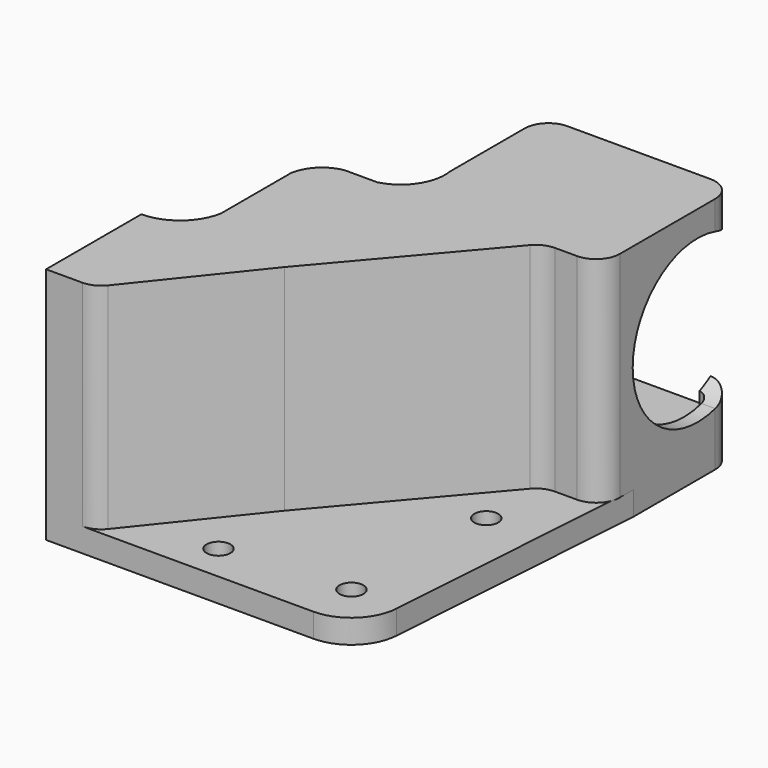
from build123d import *

# Parameters (mm, degrees)
F1_DEPTH    = 57.15
F2_T        = 3.683
F2_T3_DEPTH = 64.516
F4_DEPTH    = 25.4
F6_DEPTH    = 6.35
F7_R        = 3.175
F8_DEPTH    = 25.4
F10_DEPTH   = 56.642


# Not quite as in the source:
# - a shell that OpenCascade refuses in one call is made with other operations: the cavity is built on its own and cut out


with BuildPart() as f1:
    # F0 (on Top) → F1 (new body)
    with BuildSketch(Plane.XY):
        with BuildLine():
            ThreePointArc((33.7229068752, -2.2373507569), (35.8958962, -0.5864150612), (38.5611520326, 0))
            Line((38.5611520326, 0), (44.45, 0))
            ThreePointArc((44.45, 0), (48.9401280605, 1.8598719395), (50.8, 6.35))
            Line((50.8, 6.35), (50.8, 38.1))
            ThreePointArc((50.8, 38.1), (48.9401280605, 42.5901280605), (44.45, 44.45))
            Line((44.45, 44.45), (6.35, 44.45))
            ThreePointArc((6.35, 44.45), (1.8598719395, 42.5901280605), (0, 38.1))
            Line((0, 38.1), (0, 13.2369613275))
            ThreePointArc((0, 13.2369613275), (0.138072898, 11.4377303868), (0, 9.6384994461))
            ThreePointArc((0, 9.6384994461), (-2.9389427728, 3.4941811086), (-8.7853716686, 0))
            Line((-8.7853716686, 0), (-17.4601711333, 0))
            ThreePointArc((-17.4601711333, 0), (-22.6964673635, -2.6732403398), (-25.4, -7.893960923))
            Line((-25.4, -7.893960923), (-25.4, -31.2883965671))
            ThreePointArc((-25.4, -31.2883965671), (-29.8218894142, -38.9045945069), (-38.1, -41.91))
            Line((-38.1, -41.91), (-38.1, -73.66))
            Line((-38.1, -73.66), (-28.4519677815, -73.66))
            ThreePointArc((-28.4519677815, -73.66), (-25.7012193429, -73.0332755505), (-23.4934508416, -71.276813552))
            Line((-23.4934508416, -71.276813552), (0, -41.91))
            Line((0, -41.91), (33.7229068752, -2.2373507569))
        make_face()
    extrude(amount=F1_DEPTH)

    # F2: shell of thickness 3.683, made by hand


with BuildPart() as f2_core1:
    # F2_t2: copy of F1
    add(f1.part)

    # the walls: a layer under each face that stays
    f2_faces = [f2_core1.faces().sort_by_distance(p)[0] for p in [
        (35.8958962, -0.5864150612, 28.575),
        (6.35, -14.605, 57.15),
        (-11.7467254208, -56.593406776, 28.575),
        (-25.7012193429, -73.0332755505, 28.575),
        (-33.2759838908, -73.66, 28.575),
        (48.9401280605, 42.5901280605, 28.575),
        (50.8, 22.225, 28.575),
        (48.9401280605, 1.8598719395, 28.575),
        (6.35, -14.605, 0),
        (41.5055760163, 0, 28.575),
        (16.8614534376, -22.0736753784, 28.575),
    ]]
    thicken(f2_faces, amount=-F2_T, mode=Mode.SUBTRACT)

    # F2_s4 → F2_t3 (cut)
    with BuildSketch(Plane.XY.offset(-3.683)):
        Polygon((0.0568212202, -41.9568608842), (-2.8759398252, -39.6092481399), (-2.8416905769, -39.5664365795), (-2.8061821913, -39.524663439), align=None)
    extrude(amount=F2_T3_DEPTH, mode=Mode.SUBTRACT)


with BuildPart() as f1_1:
    add(f1.part)

    # what is left inside the walls is the cavity
    f2_cavity = [f2_core1.part.solids().sort_by_distance(p)[0] for p in [
        (15.160625, 19.021778, 3.71983),
    ]]
    add(f2_cavity, mode=Mode.SUBTRACT)

    # F3 (on face) → F4 (cut)
    with BuildSketch(Plane.YZ.offset(50.8)):
        with BuildLine():
            ThreePointArc((38.1, 7.9580365134), (49.4216390683, 15.7128126042), (53.7828262711, 28.7241964505))
            ThreePointArc((53.7828262711, 28.7241964505), (49.4216390683, 41.7355802968), (38.1, 49.4903563877))
            Line((38.1, 49.4903563877), (38.1, 7.9580365134))
        make_face()
        with BuildLine():
            Line((38.1, 7.9580365134), (38.1, 49.4903563877))
            ThreePointArc((38.1, 49.4903563877), (10.6028262711, 28.7241964505), (38.1, 7.9580365134))
        make_face()
    extrude(amount=-F4_DEPTH, mode=Mode.SUBTRACT)

    # F5 (on face) → F6 (join)
    with BuildSketch(Plane(origin=(0, 0, 0), x_dir=(1, 0, 0), z_dir=(0, 0, -1))):
        with BuildLine():
            Line((33.1074998051, 73.66), (-28.4519677815, 73.66))
            ThreePointArc((-28.4519677815, 73.66), (-25.7012193429, 73.0332755505), (-23.4934508416, 71.276813552))
            Line((-23.4934508416, 71.276813552), (0, 41.91))
            Line((0, 41.91), (33.7229068752, 2.2373507569))
            ThreePointArc((33.7229068752, 2.2373507569), (35.8958962, 0.5864150612), (38.5611520326, 0))
            Line((38.5611520326, 0), (44.45, 0))
            ThreePointArc((44.45, 0), (47.9823010709, -1.0731307441), (50.3207058028, -3.9298112931))
            Line((50.3207058028, -3.9298112931), (45.77730068, 61.8352975433))
            ThreePointArc((45.77730068, 61.8352975433), (41.7727672909, 70.2445645778), (33.1074998051, 73.66))
        make_face()
        with BuildLine():
            Line((-28.4519677815, 73.66), (-38.1, 73.66))
            Line((-38.1, 73.66), (-38.1, 41.91))
            ThreePointArc((-38.1, 41.91), (-29.7548118209, 38.9847975987), (-25.4, 31.2883965671))
            Line((-25.4, 31.2883965671), (-25.4, 7.893960923))
            ThreePointArc((-25.4, 7.893960923), (-22.5976268538, 2.7726551632), (-17.4601711333, 0))
            Line((-17.4601711333, 0), (-8.7853716686, 0))
            ThreePointArc((-8.7853716686, 0), (-1.8289491462, -4.9169285395), (0, -13.2369613275))
            Line((0, -13.2369613275), (0, -38.1))
            ThreePointArc((0, -38.1), (1.8598719395, -42.5901280605), (6.35, -44.45))
            Line((6.35, -44.45), (44.45, -44.45))
            ThreePointArc((44.45, -44.45), (48.9401280605, -42.5901280605), (50.8, -38.1))
            Line((50.8, -38.1), (50.8, -10.8675230294))
            Line((50.8, -10.8675230294), (50.3207058028, -3.9298112931))
            ThreePointArc((50.3207058028, -3.9298112931), (47.9823010709, -1.0731307441), (44.45, 0))
            Line((44.45, 0), (38.5611520326, 0))
            ThreePointArc((38.5611520326, 0), (35.8958962, 0.5864150612), (33.7229068752, 2.2373507569))
            Line((33.7229068752, 2.2373507569), (0, 41.91))
            Line((0, 41.91), (-23.4934508416, 71.276813552))
            ThreePointArc((-23.4934508416, 71.276813552), (-25.7012193429, 73.0332755505), (-28.4519677815, 73.66))
        make_face()
    extrude(amount=F6_DEPTH)

    # F7 (on face) → F8 (cut)
    with BuildSketch(Plane.XY):
        with Locations((0, -63.8569965959)):
            Circle(F7_R)
        with Locations((33.1074998051, -60.96)):
            Circle(F7_R)
        with Locations((34.9028557539, -18.2985700667)):
            Circle(F7_R)
    extrude(amount=-F8_DEPTH, mode=Mode.SUBTRACT)

    # F9 (on face) → F10 (join)
    with BuildSketch(Plane.XY.offset(57.15)):
        with BuildLine():
            Line((-9.8974186925, -28.5147787669), (-13.1322266534, -52.4904169142))
            Line((-13.1322266534, -52.4904169142), (23.2126582414, -8.8060172275))
            Line((23.2126582414, -8.8060172275), (-1.8316966669, -18.3445471934))
            ThreePointArc((-1.8316966669, -18.3445471934), (-7.2620315182, -22.3213661397), (-9.8974186925, -28.5147787669))
        make_face()
        with BuildLine():
            Line((-28.4519677815, -65.1904169142), (-28.4519677815, -67.31))
            Line((-28.4519677815, -67.31), (-27.7152992785, -69.8403045535))
            Line((-27.7152992785, -69.8403045535), (-13.1322266534, -52.4904169142))
            Line((-13.1322266534, -52.4904169142), (-15.7519677815, -52.4904169142))
            ThreePointArc((-15.7519677815, -52.4904169142), (-24.7322239026, -56.2101607932), (-28.4519677815, -65.1904169142))
        make_face()
    extrude(amount=-F10_DEPTH)


solid = f1_1.part
